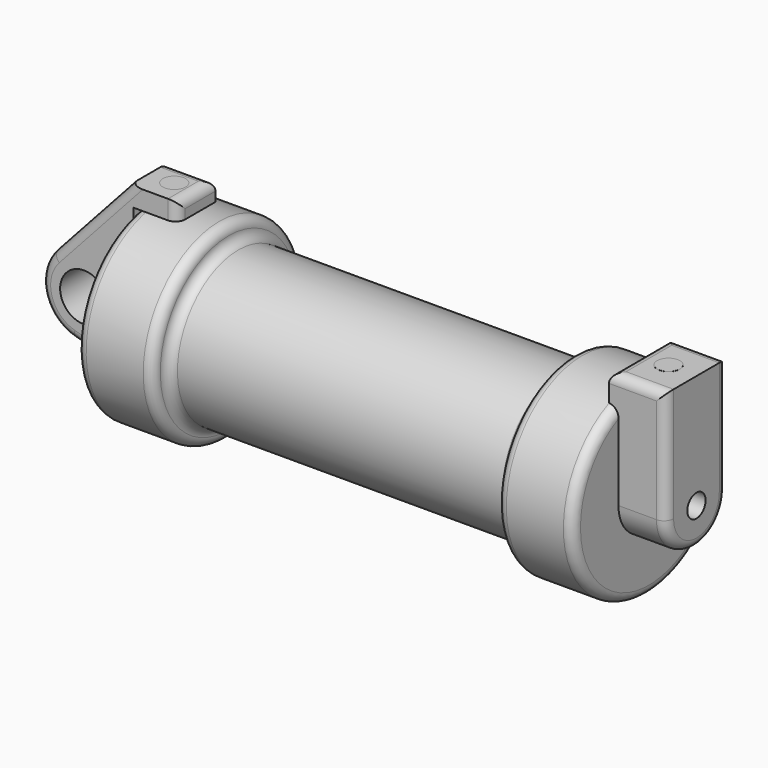
from build123d import *

# Parameters (mm, degrees)
F0_W     = 5.842
F0_H     = 12.7
F0_R     = 3.175
F2_DEPTH = 3.175
F3_R     = 1.524
F4_DEPTH = 6.35
F5_DEPTH = 1.27
F6_R     = 1.524
F7_DEPTH = 17.78
F8_DEPTH = 10.414
F9_R     = 1.26999
F10_R    = 1.26999
F11_R    = 1.27
F12_R    = 1.27


# Not quite as in the source:
# - a fillet or chamfer is up to 0.001 mm smaller than in the source, because OpenCascade refuses the exact size


with BuildPart() as f1:
    # F0 (on Front) → F1 (revolve)
    with BuildSketch(Plane.XZ):
        Polygon((5.842, 12.7), (5.842, 0), (66.294, 0), (66.294, 12.7), (56.134, 12.7), (56.134, 10.16), (10.16, 10.16), (10.16, 12.7), align=None)
        with Locations((2.921, 6.35)):
            Rectangle(F0_W, F0_H)
    revolve(axis=Axis((33.147, 0, 0), (-1, 0, 0)))

    # F3 (on face) → F4 (join)
    with BuildSketch(Plane.YZ.offset(66.294)):
        with BuildLine():
            ThreePointArc((-5.08, 11.6397422652), (0, 12.7), (5.08, 11.6397422652))
            Line((5.08, 11.6397422652), (5.08, 15.24))
            Line((5.08, 15.24), (-5.08, 15.2266876324))
            Line((-5.08, 15.2266876324), (-5.08, 11.6397422652))
        make_face()
        with BuildLine():
            ThreePointArc((-5.08, 0), (0, 5.08), (5.08, 0))
            Line((5.08, 0), (5.08, 11.6397422652))
            ThreePointArc((5.08, 11.6397422652), (0, 12.7), (-5.08, 11.6397422652))
            Line((-5.08, 11.6397422652), (-5.08, 0))
        make_face()
        with BuildLine():
            ThreePointArc((-5.08, 0), (0, -5.08), (5.08, 0))
            ThreePointArc((5.08, 0), (0, 5.08), (-5.08, 0))
        make_face()
        Circle(F3_R, mode=Mode.SUBTRACT)
    extrude(amount=F4_DEPTH)

    # F5 (add): a face of the model
    f5_faces = [f1.faces().sort_by_distance(p)[0] for p in [
        (66.294, 0.0039127163, 13.7759032878),
    ]]
    extrude(f5_faces, amount=F5_DEPTH)

    # F9 (radius 1.27 in the source; OpenCascade refuses exactly that, so slightly less here)
    f9_edges = [f1.edges().sort_by_distance(p)[0] for p in [
        (10.16, 0, -12.7),
        (0, 0, -12.7),
        (5.08, 0, 12.7),
        (10.16, 0, -10.16),
    ]]
    fillet(f9_edges, radius=F9_R)

    # F10 (radius 1.27 in the source; OpenCascade refuses exactly that, so slightly less here)
    f10_edges = [f1.edges().sort_by_distance(p)[0] for p in [
        (56.134, 0, -12.7),
        (56.134, 0, -10.16),
        (66.294, 0, -12.7),
    ]]
    fillet(f10_edges, radius=F10_R)

    # F12
    f12_edges = [f1.edges().sort_by_distance(p)[0] for p in [
        (72.644, 0, -5.08),
        (72.644, -5.08, 7.613344),
        (68.834, -5.08, 15.226688),
        (68.834, 5.08, 15.24),
        (65.024, 0, 15.233344),
    ]]
    fillet(f12_edges, radius=F12_R)


with BuildPart() as f2:
    # F0 (on Front) → F2 (new body, symmetric)
    with BuildSketch(Plane.XZ):
        with BuildLine():
            ThreePointArc((-8.1826630726, -5.5069827884), (-3.1957909266, -4.5493385486), (-0.9398, 0))
            ThreePointArc((-0.9398, 0), (-4.5919612295, 5.3297205562), (-10.8806298187, 3.8475430269))
            ThreePointArc((-10.8806298187, 3.8475430269), (-12.1459778134, -1.5837270034), (-8.1826630726, -5.5069827884))
        make_face()
        with Locations((-6.6548, 0)):
            Circle(F0_R, mode=Mode.SUBTRACT)
        with BuildLine():
            Line((5.842, 0), (0, 0))
            Line((0, 0), (-0.9398, 0))
            ThreePointArc((-0.9398, 0), (-3.1957909266, -4.5493385486), (-8.1826630726, -5.5069827884))
            Line((-8.1826630726, -5.5069827884), (5.842, -9.398))
            Line((5.842, -9.398), (5.842, 0))
        make_face()
        with BuildLine():
            Line((-0.9398, 0), (0, 0))
            Line((0, 0), (0, 12.7))
            Line((0, 12.7), (5.842, 12.7))
            Line((5.842, 12.7), (5.842, 15.24))
            Line((5.842, 15.24), (-0.508, 15.24))
            Line((-0.508, 15.24), (-10.8806298187, 3.8475430269))
            ThreePointArc((-10.8806298187, 3.8475430269), (-4.5919612295, 5.3297205562), (-0.9398, 0))
        make_face()
    extrude(amount=F2_DEPTH, both=True)

    # F11
    f11_edges = [f2.edges().sort_by_distance(p)[0] for p in [
        (-12.145978, -3.175, -1.583727),
        (-5.694315, 3.175, 9.543772),
        (5.842, -3.175, 13.97),
        (2.667, 3.175, 15.24),
        (5.842, 0, 15.24),
    ]]
    fillet(f11_edges, radius=F11_R)


with BuildPart() as f7:
    # F6 (on face) → F7 (new body)
    with BuildSketch(Plane.XY.offset(15.24)):
        with Locations((2.8348624219, 0.0535906694)):
            Circle(F6_R)
    extrude(amount=-F7_DEPTH)


with BuildPart() as f8:
    # F6 (on face) → F8 (new body)
    with BuildSketch(Plane.XY.offset(15.24)):
        with Locations((68.7882303587, 0.1481550013)):
            Circle(F6_R)
    extrude(amount=-F8_DEPTH)


solid = Compound([f1.part, f2.part, f7.part, f8.part])
